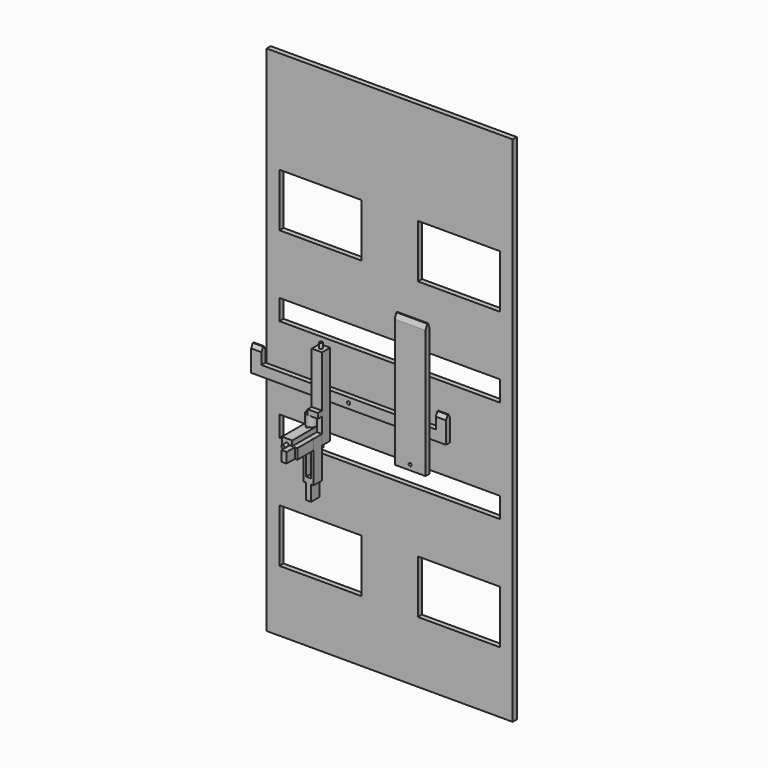
from build123d import *

# Parameters (mm, degrees)
F0_R       = 1.5
F1_DEPTH   = 5
F2_SIZE2   = 2
F2_SIZE    = 4
F2_2_SIZE2 = 2
F2_2_SIZE  = 4
F4_W       = 30
F4_H       = 130
F4_R       = 1.5
F5_DEPTH   = 5
F6_SIZE2   = 2
F6_SIZE    = 5
F6_2_SIZE2 = 2
F6_2_SIZE  = 5
F7_W       = 10
F7_H       = 10
F8_DEPTH   = 30
F9_R       = 1.5
F10_DEPTH  = 5
F11_R      = 1.5
F12_DEPTH  = 5
F14_DEPTH  = 10
F15_R      = 1.5
F16_DEPTH  = 5
F18_R      = 1.5
F19_DEPTH  = 135.001
F17_W      = 5
F17_H      = 10
F20_DEPTH  = 10
F21_W      = 5
F21_H      = 30
F22_DEPTH  = 10
F23_W      = 240
F23_H      = 500
F23_W_2    = 80
F23_H_2    = 52
F23_W_3    = 215
F23_H_3    = 20
F24_DEPTH  = 5
F25_R      = 1.5
F26_DEPTH  = 5
F27_R      = 2
F28_DEPTH  = 5
F31_R      = 5
F31_R_2    = 3.5
F32_DEPTH  = 15


with BuildPart() as f1:
    # F0 (on Front) → F1 (new body)
    with BuildSketch(Plane.XZ):
        Polygon((-95, 0), (0, 0), (95, 0), (95, 25), (85, 25), (85, 10), (0, 10), (-85, 10), (-85, 25), (-95, 25), align=None)
        with Locations((0, 5)):
            Circle(F0_R, mode=Mode.SUBTRACT)
    extrude(amount=F1_DEPTH)

    # F2
    f2_edges = [f1.edges().sort_by_distance(p)[0] for p in [
        (90, -5, 25),
        (-90, -5, 25),
    ]]
    f2_side = f1.faces().sort_by_distance((0, -5, 6.71004))[0]
    chamfer(f2_edges, length=F2_SIZE, length2=F2_SIZE2, reference=f2_side)

    # F2#2
    f2_2_edges = [f1.edges().sort_by_distance(p)[0] for p in [
        (90, 0, 25),
        (-90, 0, 25),
    ]]
    f2_2_side = f1.faces().sort_by_distance((0, 0, 6.71004))[0]
    chamfer(f2_2_edges, length=F2_2_SIZE, length2=F2_2_SIZE2, reference=f2_2_side)


with BuildPart() as f1_1:
    # F3: moved
    add(f1.part.moved(Location((0, 50, 0))))


with BuildPart() as f5:
    # F4 (on Front) → F5 (new body)
    with BuildSketch(Plane.XZ):
        with Locations((0, 65)):
            Rectangle(F4_W, F4_H)
        with Locations((0, 5)):
            Circle(F4_R, mode=Mode.SUBTRACT)
    extrude(amount=F5_DEPTH)

    # F6
    f6_edges = [f5.edges().sort_by_distance(p)[0] for p in [
        (0, -5, 130),
    ]]
    f6_side = f5.faces().sort_by_distance((0, -5, 65.108945))[0]
    chamfer(f6_edges, length=F6_SIZE, length2=F6_SIZE2, reference=f6_side)

    # F6#2
    f6_2_edges = [f5.edges().sort_by_distance(p)[0] for p in [
        (0, 0, 130),
    ]]
    f6_2_side = f5.faces().sort_by_distance((0, 0, 65.108945))[0]
    chamfer(f6_2_edges, length=F6_2_SIZE, length2=F6_2_SIZE2, reference=f6_2_side)


with BuildPart() as f8:
    # F7 (on Front) → F8 (new body)
    with BuildSketch(Plane.XZ):
        Rectangle(F7_W, F7_H)
    extrude(amount=F8_DEPTH)

    # F9 (on face) → F10 (join)
    with BuildSketch(Plane.XZ.offset(30)):
        Circle(F9_R)
    extrude(amount=F10_DEPTH)

    # F11 (on face) → F12 (join)
    with BuildSketch(Plane(origin=(0, 0, 0), x_dir=(-1, 0, 0), z_dir=(0, 1, 0))):
        Circle(F11_R)
    extrude(amount=F12_DEPTH)

    # F18 (on face) → F19 (cut, through all)
    with BuildSketch(Plane(origin=(0, 0, -5), x_dir=(1, 0, 0), z_dir=(0, 0, -1))):
        with Locations((0, 5)):
            Circle(F18_R)
    extrude(amount=-F19_DEPTH, mode=Mode.SUBTRACT)


with BuildPart() as f14:
    # F13 (on Right) → F14 (new body)
    with BuildSketch(Plane.YZ):
        Polygon((10, 70), (0, 70), (0, 20), (-5, 20), (-5, 15), (0, 15), (0, 0), (-30, 0), (-30, -10), (10, -10), align=None)
    extrude(amount=F14_DEPTH)

    # F15 (on face) → F16 (join)
    with BuildSketch(Plane.XY.offset(70)):
        with Locations((5, 5)):
            Circle(F15_R)
    extrude(amount=F16_DEPTH)

    # F17 (on face) → F20 (join)
    with BuildSketch(Plane.XZ.offset(30)):
        with Locations((5, -5)):
            Rectangle(F17_W, F17_H)
    extrude(amount=F20_DEPTH)

    # F27 (on face) → F28 (join)
    with BuildSketch(Plane(origin=(0, 0, -10), x_dir=(1, 0, 0), z_dir=(0, 0, -1))):
        with Locations((5, -5)):
            Circle(F27_R)
    extrude(amount=F28_DEPTH)


with BuildPart() as f22:
    # F21 (on Front) → F22 (new body)
    with BuildSketch(Plane.XZ):
        Polygon((10, 0), (0, 0), (0, -40), (2.5, -40), (2.5, -55), (7.5, -55), (7.5, -40), (10, -40), align=None)
        with Locations((5, -20)):
            Rectangle(F21_W, F21_H, mode=Mode.SUBTRACT)
    extrude(amount=F22_DEPTH)


with BuildPart() as f24:
    # F23 (on Front) → F24 (new body)
    with BuildSketch(Plane.XZ):
        Rectangle(F23_W, F23_H)
        with Locations((-67.5, -164)):
            Rectangle(F23_W_2, F23_H_2, mode=Mode.SUBTRACT)
        with Locations((67.5, -164)):
            Rectangle(F23_W_2, F23_H_2, mode=Mode.SUBTRACT)
        with Locations((0, -70)):
            Rectangle(F23_W_3, F23_H_3, mode=Mode.SUBTRACT)
        with Locations((-67.5, 124)):
            Rectangle(F23_W_2, F23_H_2, mode=Mode.SUBTRACT)
        with Locations((0, 30)):
            Rectangle(F23_W_3, F23_H_3, mode=Mode.SUBTRACT)
        with Locations((67.5, 124)):
            Rectangle(F23_W_2, F23_H_2, mode=Mode.SUBTRACT)
    extrude(amount=F24_DEPTH)

    # F25 (on face) → F26 (cut)
    with BuildSketch(Plane(origin=(0, 0, -250), x_dir=(1, 0, 0), z_dir=(0, 0, -1))):
        with Locations((0, 2.5)):
            Circle(F25_R)
    extrude(amount=-F26_DEPTH, mode=Mode.SUBTRACT)


with BuildPart() as f24_1:
    # F29: moved
    add(f24.part.moved(Location((0, 100, 0))))


with BuildPart() as f5_1:
    # F30: moved
    add(f5.part.moved(Location((100, 0, 0))))


with BuildPart() as f32:
    # F31 (on Top) → F32 (new body)
    with BuildSketch(Plane.XY):
        Circle(F31_R)
        Circle(F31_R_2, mode=Mode.SUBTRACT)
    extrude(amount=F32_DEPTH)


solid = Compound([f1_1.part, f8.part, f14.part, f22.part, f24_1.part, f5_1.part, f32.part])
